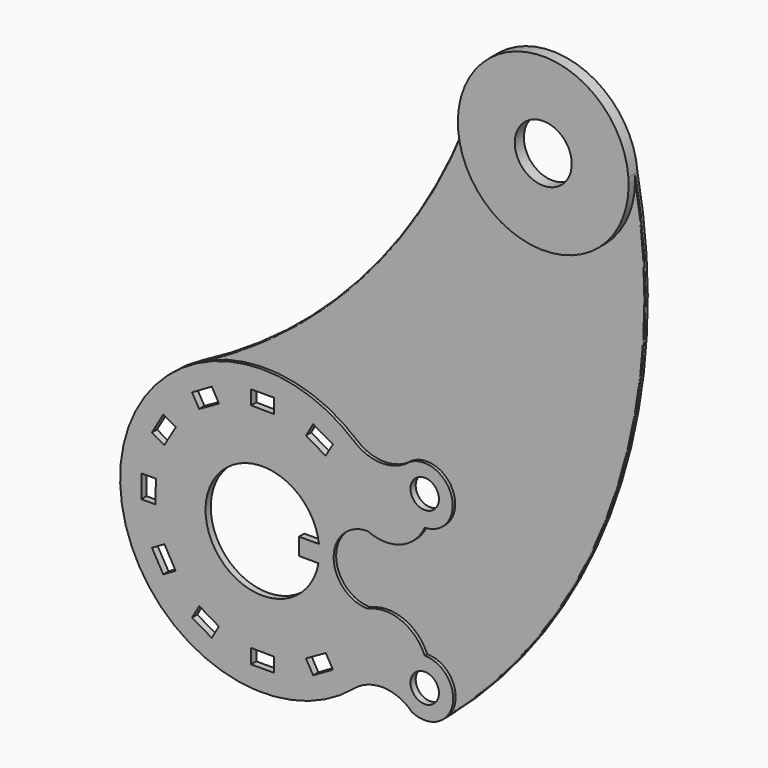
from build123d import *

# Parameters (mm, degrees)
F0_R        = 5
F1_DEPTH    = 2.3
F2_DEPTH    = 1.2
F0_R_2      = 10
F3_DEPTH    = 4
F4_T4_ANGLE = 61.2690035525
F4_S5_R     = 30
F4_T6_DEPTH = 114
F4_S7_R     = 10
F4_T8_DEPTH = 114
F5_T4_ANGLE = 41.074053593
F5_S5_R     = 30
F5_T6_DEPTH = 82
F5_S7_R     = 50
F5_T8_DEPTH = 82


# Not quite as in the source:
# - a fillet or chamfer that OpenCascade refuses, or shapes differently, is made with other operations: its cross-section is extruded or revolved along the edge and cut away or added


with BuildPart() as f1:
    # F0 (on Front) → F1 (new body)
    with BuildSketch(Plane.XZ):
        with BuildLine():
            ThreePointArc((51.6923076923, 38.1603592456), (42, 34.6084670192), (32.3076923077, 38.1603592456))
            ThreePointArc((32.3076923077, 38.1603592456), (5.5214165196, 49.6942044872), (-23.1433206058, 44.3214024072))
            ThreePointArc((-23.1433206058, 44.3214024072), (-41.4946584334, -27.8961166023), (32.3076923077, -38.1603592456))
            ThreePointArc((32.3076923077, -38.1603592456), (42.5952420348, -34.6202821085), (52.5696525848, -38.9650444383))
            ThreePointArc((52.5696525848, -38.9650444383), (58.5892524469, -39.8729061912), (64.0198786028, -37.1218891035))
            ThreePointArc((64.0198786028, -37.1218891035), (66.2525372476, -26.2065115681), (57, -20))
            ThreePointArc((57, -20), (48.6934276496, -11.7664308759), (37, -12))
            ThreePointArc((37, -12), (25, 0), (37, 12))
            ThreePointArc((37, 12), (48.5892751146, 11.6008362262), (57, 19.5839644541))
            ThreePointArc((57, 19.5839644541), (66.4476997873, 32.3298447331), (51.6923076923, 38.1603592456))
        make_face()
        Polygon((-15.306354845, -34.5113842702), (-17.806354845, -38.8415112891), (-24.7345580753, -34.8415112891), (-22.1933950155, -30.4400877594), align=None, mode=Mode.SUBTRACT)
        Polygon((-30.5113842702, -22.2345580753), (-34.8415112891, -24.7345580753), (-38.8415112891, -17.806354845), (-34.4400877594, -15.2651917853), align=None, mode=Mode.SUBTRACT)
        Polygon((-37.5409129203, -4), (-42.5409129203, -4), (-42.5409129203, 4), (-37.4585868008, 4), align=None, mode=Mode.SUBTRACT)
        Polygon((3.9995764343, -37.5409085614), (3.9995764343, -42.5409129203), (-4, -42.5409129203), (-4, -37.4585868008), align=None, mode=Mode.SUBTRACT)
        Polygon((22.2341890772, -30.5115922782), (24.7341890772, -34.8417192971), (17.8063526656, -38.8415075143), (15.2651917853, -34.4400877594), align=None, mode=Mode.SUBTRACT)
        with BuildLine():
            Line((19.8513816884, 2.433648508), (12.8513816884, 2.433648508))
            Line((12.8513816884, 2.433648508), (12.8513816884, -3.566351492))
            Line((12.8513816884, -3.566351492), (19.679459775, -3.566351492))
            ThreePointArc((19.679459775, -3.566351492), (-19.9917947344, 0.572837934), (19.8513816884, 2.433648508))
        make_face(mode=Mode.SUBTRACT)
        Polygon((-34.5113842702, 15.306354845), (-38.8415112891, 17.806354845), (-34.8415112891, 24.7345580753), (-30.4400877594, 22.1933950155), align=None, mode=Mode.SUBTRACT)
        Polygon((-22.2345580753, 30.5113842702), (-24.7345580753, 34.8415112891), (-17.806354845, 38.8415112891), (-15.2651917853, 34.4400877594), align=None, mode=Mode.SUBTRACT)
        Polygon((15.306354845, 34.5113842702), (17.806354845, 38.8415112891), (24.7345580753, 34.8415112891), (22.1933950155, 30.4400877594), align=None, mode=Mode.SUBTRACT)
        Polygon((-4, 37.5409129203), (-4, 42.5409129203), (4, 42.5409129203), (4, 37.4585868008), align=None, mode=Mode.SUBTRACT)
        with Locations((57, -30)):
            Circle(F0_R, mode=Mode.SUBTRACT)
        with Locations((57, 30)):
            Circle(F0_R, mode=Mode.SUBTRACT)
    extrude(amount=F1_DEPTH)

    # F0 (on Front) → F2 (join)
    with BuildSketch(Plane.XZ):
        with BuildLine():
            ThreePointArc((-23.1433206058, 44.3214024072), (5.5214165196, 49.6942044872), (32.3076923077, 38.1603592456))
            ThreePointArc((32.3076923077, 38.1603592456), (42, 34.6084670192), (51.6923076923, 38.1603592456))
            ThreePointArc((51.6923076923, 38.1603592456), (66.4476997873, 32.3298447331), (57, 19.5839644541))
            ThreePointArc((57, 19.5839644541), (48.5892751146, 11.6008362262), (37, 12))
            ThreePointArc((37, 12), (25, 0), (37, -12))
            ThreePointArc((37, -12), (48.6934276496, -11.7664308759), (57, -20))
            ThreePointArc((57, -20), (66.2525372476, -26.2065115681), (64.0198786028, -37.1218891035))
            ThreePointArc((64.0198786028, -37.1218891035), (122.4330747785, 48.7493192224), (129.9089599648, 152.3354044245))
            ThreePointArc((129.9089599648, 152.3354044245), (129.977231351, 151.1685891188), (130, 150))
            ThreePointArc((130, 150), (101.1913208393, 120.0236634217), (70.0946163561, 147.6192377033))
            ThreePointArc((70.0946163561, 147.6192377033), (32.7491957463, 87.5998980678), (-23.1433206058, 44.3214024072))
        make_face()
    extrude(amount=F2_DEPTH)

    # F0 (on Front) → F3 (join)
    with BuildSketch(Plane.XZ):
        with BuildLine():
            ThreePointArc((129.9089599648, 152.3354044245), (97.6419159614, 179.9071804032), (70.0946163561, 147.6192377033))
            ThreePointArc((70.0946163561, 147.6192377033), (101.1913208393, 120.0236634217), (130, 150))
            ThreePointArc((130, 150), (129.977231351, 151.1685891188), (129.9089599648, 152.3354044245))
        make_face()
        with Locations((100, 150)):
            Circle(F0_R_2, mode=Mode.SUBTRACT)
    extrude(amount=F3_DEPTH)

    # F4: fillet of radius 0.25 on 1 edges, made by hand


with BuildPart() as f4_tool2:
    # F4_s3 → F4_t4 (revolve)
    with BuildSketch(Plane(origin=(17.0947609574, 0, 14.2583854823), x_dir=(0, 1, 0), z_dir=(-0.7679394892, 0, -0.6405223969))):
        with BuildLine():
            ThreePointArc((-1.2, 69.2879529885), (-1.1267766953, 69.4647296838), (-0.95, 69.5379529885))
            Line((-0.95, 69.5379529885), (-1.2, 69.5379529885))
            Line((-1.2, 69.5379529885), (-1.2, 69.2879529885))
        make_face()
    revolve(axis=Axis((-66.469102104, -1.2, 114.4453432197), (0, -1, 0)), revolution_arc=F4_T4_ANGLE)

    # F4_s5 → F4_t6 (cut, symmetric)
    with BuildSketch(Plane.XZ.offset(1)):
        with Locations((100, 150)):
            Circle(F4_S5_R)
    extrude(amount=F4_T6_DEPTH, both=True, mode=Mode.SUBTRACT)

    # F4_s7 → F4_t8 (cut, symmetric)
    with BuildSketch(Plane.XZ.offset(1)):
        with Locations((57, -30)):
            Circle(F4_S7_R)
    extrude(amount=F4_T8_DEPTH, both=True, mode=Mode.SUBTRACT)


with BuildPart() as f1_1:
    add(f1.part)

    # F4_t1: cut F4_tool2
    add(f4_tool2.part, mode=Mode.SUBTRACT)

    # F5: fillet of radius 0.25 on 1 edges, made by hand


with BuildPart() as f5_tool2:
    # F5_s3 → F5_t4 (revolve)
    with BuildSketch(Plane(origin=(60.0718928504, 0, 152.245866678), x_dir=(0, 1, 0), z_dir=(0.3670335308, 0, 0.9302077119))):
        with BuildLine():
            ThreePointArc((-1.2, -11.2723193897), (-1.1267766953, -11.0955426945), (-0.95, -11.0223193897))
            Line((-0.95, -11.0223193897), (-1.2, -11.0223193897))
            Line((-1.2, -11.0223193897), (-1.2, -11.2723193897))
        make_face()
    revolve(axis=Axis((-115.7166030288, -1.2, 221.6070120359), (0, 1, 0)), revolution_arc=F5_T4_ANGLE)

    # F5_s5 → F5_t6 (cut, symmetric)
    with BuildSketch(Plane.XZ.offset(1)):
        with Locations((100, 150)):
            Circle(F5_S5_R)
    extrude(amount=F5_T6_DEPTH, both=True, mode=Mode.SUBTRACT)

    # F5_s7 → F5_t8 (cut, symmetric)
    with BuildSketch(Plane.XZ.offset(1)):
        Circle(F5_S7_R)
    extrude(amount=F5_T8_DEPTH, both=True, mode=Mode.SUBTRACT)


with BuildPart() as f1_2:
    add(f1_1.part)

    # F5_t1: cut F5_tool2
    add(f5_tool2.part, mode=Mode.SUBTRACT)


solid = f1_2.part
